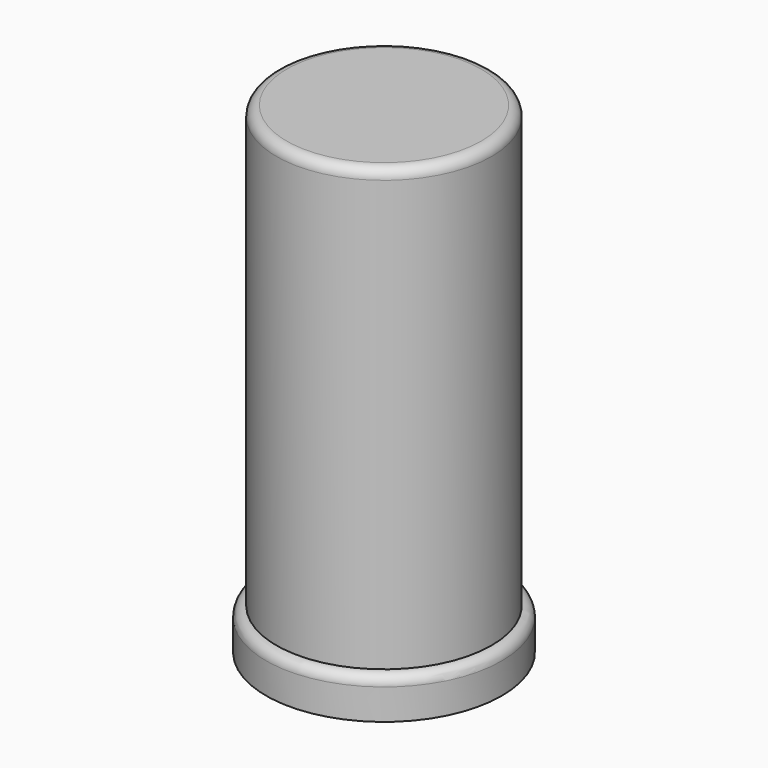
from build123d import *

# Parameters (mm, degrees)
F0_R     = 18.25625
F1_DEPTH = 6.35
F2_R     = 16.66875
F3_DEPTH = 68.2625
F4_R     = 1.58749


# Not quite as in the source:
# - a fillet or chamfer is up to 0.001 mm smaller than in the source, because OpenCascade refuses the exact size


with BuildPart() as f1:
    # F0 (on Top) → F1 (new body)
    with BuildSketch(Plane.XY):
        Circle(F0_R)
    extrude(amount=F1_DEPTH)

    # F2 (on face) → F3 (join)
    with BuildSketch(Plane.XY.offset(6.35)):
        Circle(F2_R)
    extrude(amount=F3_DEPTH)

    # F4 (radius 1.5875 in the source; OpenCascade refuses exactly that, so slightly less here)
    f4_edges = [f1.edges().sort_by_distance(p)[0] for p in [
        (-18.25625, 0, 6.35),
        (-16.66875, 0, 74.6125),
    ]]
    fillet(f4_edges, radius=F4_R)


solid = f1.part
